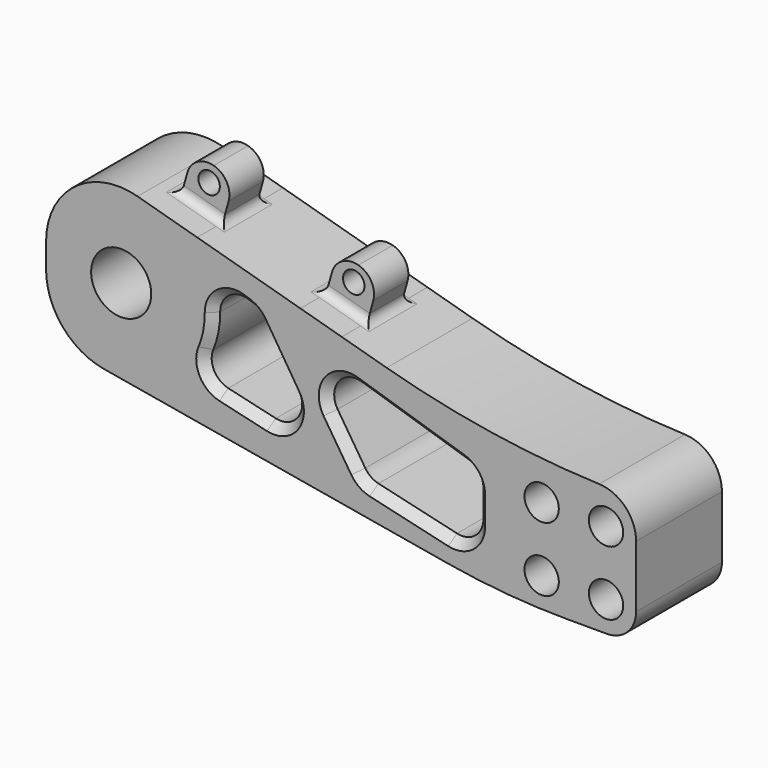
from build123d import *

# Parameters (mm, degrees)
F0_W          = 30
F0_H          = 30
F0_R          = 4
F0_R_2        = 7
F1_DEPTH      = 25
F2_R          = 16.7849194194
F3_R          = 16.2658089237
F4_R          = 212.1999742311
F5_R          = 163.8141108575
F6_R          = 8.9325901808
F7_R          = 6.7597979746
F9_DEPTH      = 25
F10_R         = 5
F11_SIZE      = 2
F13_DEPTH     = 7.5
F15_DEPTH     = 7.5
F16_T1_DEPTH  = 10
F16_T3_DEPTH  = 10
F16_T5_DEPTH  = 10
F16_T7_DEPTH  = 10
F16_T9_DEPTH  = 10
F16_T15_DEPTH = 12
F16_T19_DEPTH = 12
F16_T26_DEPTH = 12
F16_T30_DEPTH = 12
F16_T37_DEPTH = 12
F16_T41_DEPTH = 12
F16_T48_DEPTH = 12
F16_T52_DEPTH = 12
F16_T59_DEPTH = 12
F16_T63_DEPTH = 12
F16_T70_DEPTH = 12
F16_T74_DEPTH = 12
F16_T81_DEPTH = 12
F16_T85_DEPTH = 12
F16_T92_DEPTH = 12
F16_T96_DEPTH = 12
F17_R         = 2.5
F18_DEPTH     = 25
F19_R         = 4.99999


# Not quite as in the source:
# - a fillet or chamfer that OpenCascade refuses, or shapes differently, is made with other operations: its cross-section is extruded or revolved along the edge and cut away or added
# - a fillet or chamfer is up to 0.001 mm smaller than in the source, because OpenCascade refuses the exact size


with BuildPart() as f1:
    # F0 (on Front) → F1 (new body)
    with BuildSketch(Plane.XZ):
        Rectangle(F0_W, F0_H)
        with Locations((-7, -8)):
            Circle(F0_R, mode=Mode.SUBTRACT)
        with Locations((8, -8)):
            Circle(F0_R, mode=Mode.SUBTRACT)
        with Locations((-7, 7)):
            Circle(F0_R, mode=Mode.SUBTRACT)
        with Locations((8, 7)):
            Circle(F0_R, mode=Mode.SUBTRACT)
        Polygon((-15, -15), (-15, 15), (-53.5854479095, 25.8251958423), (-63.2137087554, 28.5264165077), (-87.2843608702, 35.2794681713), (-96.9126217161, 37.9806888367), (-122.4668100476, 45.1499484479), (-122.4668100476, 3.5487897694), align=None)
        with Locations((-104.9668100476, 20.1499484479)):
            Circle(F0_R_2, mode=Mode.SUBTRACT)
        Polygon((-63.2137087554, 28.5264165077), (-53.5854479095, 25.8251958423), (-50.8842272441, 35.4534566882), (-60.51248809, 38.1546773536), align=None)
        Polygon((-96.9126217161, 37.9806888367), (-87.2843608702, 35.2794681713), (-84.5831402048, 44.9077290172), (-94.2114010507, 47.6089496826), align=None)
    extrude(amount=F1_DEPTH)

    # F2
    f2_edges = [f1.edges().sort_by_distance(p)[0] for p in [
        (-122.46681, -12.5, 45.149948),
    ]]
    fillet(f2_edges, radius=F2_R)

    # F3
    f3_edges = [f1.edges().sort_by_distance(p)[0] for p in [
        (-122.46681, -12.5, 3.54879),
    ]]
    fillet(f3_edges, radius=F3_R)

    # F4
    f4_edges = [f1.edges().sort_by_distance(p)[0] for p in [
        (-15, -12.5, 15),
    ]]
    fillet(f4_edges, radius=F4_R)

    # F5
    f5_edges = [f1.edges().sort_by_distance(p)[0] for p in [
        (-15, -12.5, -15),
    ]]
    fillet(f5_edges, radius=F5_R)

    # F6
    f6_edges = [f1.edges().sort_by_distance(p)[0] for p in [
        (15, -12.5, 15),
    ]]
    fillet(f6_edges, radius=F6_R)

    # F7
    f7_edges = [f1.edges().sort_by_distance(p)[0] for p in [
        (15, -12.5, -15),
    ]]
    fillet(f7_edges, radius=F7_R)

    # F8 (on face) → F9 (cut)
    with BuildSketch(Plane.XZ.offset(25)):
        with BuildLine():
            Line((-73.9658618647, 24.2199581794), (-84.8379017791, 27.6423353583))
            ThreePointArc((-84.8379017791, 27.6423353583), (-83.7792374174, 16.8291979096), (-88.2094318459, 6.9086087616))
            Line((-88.2094318459, 6.9086087616), (-58.6424097419, 0))
            Line((-58.6424097419, 0), (-73.9658618647, 24.2199581794))
        make_face()
        Polygon((-22.1739318222, -8.5211978803), (-22.1739318222, 7.9165302277), (-63.6694356799, 20.978776738), (-48.5837496817, -2.3502991535), align=None)
    extrude(amount=-F9_DEPTH, mode=Mode.SUBTRACT)

    # F10
    f10_edges = [f1.edges().sort_by_distance(p)[0] for p in [
        (-88.209432, -12.5, 6.908609),
        (-84.837902, -12.5, 27.642335),
        (-73.965862, -12.5, 24.219958),
        (-58.64241, -12.5, 0),
        (-63.669436, -12.5, 20.978777),
        (-48.58375, -12.5, -2.350299),
        (-22.173932, -12.5, -8.521198),
        (-22.173932, -12.5, 7.91653),
    ]]
    fillet(f10_edges, radius=F10_R)

    # F11
    f11_edges = [f1.edges().sort_by_distance(p)[0] for p in [
        (-81.475167, -25, 24.42871),
        (-38.054326, -25, 12.915472),
        (-38.054326, 0, 12.915472),
        (-69.079861, 0, 16.497238),
        (-52.90778, 0, 4.336545),
        (-55.915109, 0, 15.073198),
        (-48.358225, 0, -2.029785),
        (-37.465092, 0, -4.948277),
        (-23.142397, 0, 7.206075),
        (-24.066543, 0, -6.135382),
        (-22.173932, 0, 1.015182),
        (-76.357367, 0, 24.972773),
        (-74.163675, 0, 23.962872),
        (-81.475167, 0, 24.42871),
        (-83.895301, 0, 16.17939),
        (-65.322794, 0, 4.750228),
        (-84.930719, 0, 7.951227),
        (-76.078695, 0, 4.07415),
        (-52.90778, -25, 4.336545),
        (-55.915109, -25, 15.073198),
        (-48.358225, -25, -2.029785),
        (-37.465092, -25, -4.948277),
        (-23.142397, -25, 7.206075),
        (-24.066543, -25, -6.135382),
        (-22.173932, -25, 1.015182),
        (-76.357367, -25, 24.972773),
        (-74.163675, -25, 23.962872),
        (-69.079861, -25, 16.497238),
        (-83.895301, -25, 16.17939),
        (-65.322794, -25, 4.750228),
        (-84.930719, -25, 7.951227),
        (-76.078695, -25, 4.07415),
    ]]
    chamfer(f11_edges, length=F11_SIZE)

    # F12 (on face) → F13 (cut)
    with BuildSketch(Plane.XZ.offset(25)):
        Polygon((-50.8842272441, 35.4534566882), (-60.51248809, 38.1546773536), (-63.2137087554, 28.5264165077), (-53.5854479095, 25.8251958423), align=None)
        Polygon((-87.2843608702, 35.2794681713), (-84.5831402048, 44.9077290172), (-94.2114010507, 47.6089496826), (-96.9126217161, 37.9806888367), align=None)
    extrude(amount=-F13_DEPTH, mode=Mode.SUBTRACT)

    # F14 (on face) → F15 (cut)
    with BuildSketch(Plane(origin=(0, 0, 0), x_dir=(-1, 0, 0), z_dir=(0, 1, 0))):
        Polygon((53.5854479095, 25.8251958423), (63.2137087554, 28.5264165077), (60.51248809, 38.1546773536), (50.8842272441, 35.4534566882), align=None)
        Polygon((94.2114010507, 47.6089496826), (84.5831402048, 44.9077290172), (87.2843608702, 35.2794681713), (96.9126217161, 37.9806888367), align=None)
    extrude(amount=-F15_DEPTH, mode=Mode.SUBTRACT)

    # F16: fillet of radius 2 on 8 edges, made by hand

    # F16_s2 → F16_t1 (join)
    with BuildSketch(Plane(origin=(-56.3921675224, 0, 15.8208933801), x_dir=(0, 1, 0), z_dir=(-0.9628260846, 0, 0.2701220665))):
        with BuildLine():
            ThreePointArc((-5.5, -10.3905602707), (-6.9142135624, -10.9763467084), (-7.5, -12.3905602707))
            Line((-7.5, -12.3905602707), (-7.54, -12.3905602707))
            Line((-7.54, -12.3905602707), (-7.54, -10.3505602707))
            Line((-7.54, -10.3505602707), (-5.5, -10.3505602707))
            Line((-5.5, -10.3505602707), (-5.5, -10.3905602707))
        make_face()
    extrude(amount=F16_T1_DEPTH)

    # F16_s4 → F16_t3 (join)
    with BuildSketch(Plane.XZ.offset(7.5)):
        with BuildLine():
            ThreePointArc((-51.6597957404, 25.2849517092), (-52.8632036043, 26.2309724614), (-53.0452037765, 27.7508480115))
            Line((-53.0452037765, 27.7508480115), (-53.0837168198, 27.7616528941))
            Line((-53.0837168198, 27.7616528941), (-53.6347658356, 25.7974876816))
            Line((-53.6347658356, 25.7974876816), (-51.670600623, 25.2464386658))
            Line((-51.670600623, 25.2464386658), (-51.6597957404, 25.2849517092))
        make_face()
        with BuildLine():
            ThreePointArc((-65.1393609246, 29.0666606408), (-63.6194853745, 29.248660813), (-62.6734646224, 30.4520686769))
            Line((-62.6734646224, 30.4520686769), (-62.634951579, 30.4412637942))
            Line((-62.634951579, 30.4412637942), (-63.1860005947, 28.4770985817))
            Line((-63.1860005947, 28.4770985817), (-65.1501658073, 29.0281475974))
            Line((-65.1501658073, 29.0281475974), (-65.1393609246, 29.0666606408))
        make_face()
        with BuildLine():
            ThreePointArc((-85.358708701, 34.7392240382), (-86.562116565, 35.6852447903), (-86.7441167371, 37.2051203404))
            Line((-86.7441167371, 37.2051203404), (-86.7826297805, 37.2159252231))
            Line((-86.7826297805, 37.2159252231), (-87.3336787962, 35.2517600105))
            Line((-87.3336787962, 35.2517600105), (-85.3695135837, 34.7007109948))
            Line((-85.3695135837, 34.7007109948), (-85.358708701, 34.7392240382))
        make_face()
        with BuildLine():
            ThreePointArc((-98.8382738853, 38.5209329698), (-97.3183983352, 38.7029331419), (-96.372377583, 39.9063410059))
            Line((-96.372377583, 39.9063410059), (-96.3338645396, 39.8955361232))
            Line((-96.3338645396, 39.8955361232), (-96.8849135554, 37.9313709106))
            Line((-96.8849135554, 37.9313709106), (-98.8490787679, 38.4824199264))
            Line((-98.8490787679, 38.4824199264), (-98.8382738853, 38.5209329698))
        make_face()
    extrude(amount=F16_T3_DEPTH)

    # F16_s6 → F16_t5 (join)
    with BuildSketch(Plane(origin=(-66.0204283683, 0, 18.5221140456), x_dir=(0, 1, 0), z_dir=(0.9628260846, 0, -0.2701220665))):
        with BuildLine():
            ThreePointArc((-19.5, 10.3905602707), (-18.0857864376, 10.9763467084), (-17.5, 12.3905602707))
            Line((-17.5, 12.3905602707), (-17.46, 12.3905602707))
            Line((-17.46, 12.3905602707), (-17.46, 10.3505602707))
            Line((-17.46, 10.3505602707), (-19.5, 10.3505602707))
            Line((-19.5, 10.3505602707), (-19.5, 10.3905602707))
        make_face()
    extrude(amount=F16_T5_DEPTH)

    # F16_s8 → F16_t7 (join)
    with BuildSketch(Plane(origin=(-99.7193413289, 0, 27.9763863745), x_dir=(0, 1, 0), z_dir=(0.9628260846, 0, -0.2701220665))):
        with BuildLine():
            ThreePointArc((-19.5, 10.3905602707), (-18.0857864376, 10.9763467084), (-17.5, 12.3905602707))
            Line((-17.5, 12.3905602707), (-17.46, 12.3905602707))
            Line((-17.46, 12.3905602707), (-17.46, 10.3505602707))
            Line((-17.46, 10.3505602707), (-19.5, 10.3505602707))
            Line((-19.5, 10.3505602707), (-19.5, 10.3905602707))
        make_face()
    extrude(amount=F16_T7_DEPTH)

    # F16_s10 → F16_t9 (join)
    with BuildSketch(Plane(origin=(-90.091080483, 0, 25.2751657091), x_dir=(0, 1, 0), z_dir=(-0.9628260846, 0, 0.2701220665))):
        with BuildLine():
            ThreePointArc((-5.5, -10.3905602707), (-6.9142135624, -10.9763467084), (-7.5, -12.3905602707))
            Line((-7.5, -12.3905602707), (-7.54, -12.3905602707))
            Line((-7.54, -12.3905602707), (-7.54, -10.3505602707))
            Line((-7.54, -10.3505602707), (-5.5, -10.3505602707))
            Line((-5.5, -10.3505602707), (-5.5, -10.3905602707))
        make_face()
    extrude(amount=F16_T9_DEPTH)


with BuildPart() as f16_tool13:
    # F16_s14 → F16_t15 (new body)
    with BuildSketch(Plane.XZ.offset(5.5)):
        with BuildLine():
            ThreePointArc((-51.6597957404, 25.2849517092), (-52.8632036043, 26.2309724614), (-53.0452037765, 27.7508480115))
            Line((-53.0452037765, 27.7508480115), (-53.0837168198, 27.7616528941))
            Line((-53.0837168198, 27.7616528941), (-53.6347658356, 25.7974876816))
            Line((-53.6347658356, 25.7974876816), (-51.670600623, 25.2464386658))
            Line((-51.670600623, 25.2464386658), (-51.6597957404, 25.2849517092))
        make_face()
    extrude(amount=F16_T15_DEPTH)

    split(bisect_by=Plane.XZ.offset(7.5), keep=Keep.BOTTOM)


with BuildPart() as f16_tool17:
    # F16_s18 → F16_t19 (new body)
    with BuildSketch(Plane(origin=(-54.4665153532, 0, 15.2806492471), x_dir=(0, 1, 0), z_dir=(-0.9628260846, 0, 0.2701220665))):
        with BuildLine():
            ThreePointArc((-5.5, -10.3905602707), (-6.9142135624, -10.9763467084), (-7.5, -12.3905602707))
            Line((-7.5, -12.3905602707), (-7.54, -12.3905602707))
            Line((-7.54, -12.3905602707), (-7.54, -10.3505602707))
            Line((-7.54, -10.3505602707), (-5.5, -10.3505602707))
            Line((-5.5, -10.3505602707), (-5.5, -10.3905602707))
        make_face()
    extrude(amount=F16_T19_DEPTH)

    split(bisect_by=Plane(origin=(-56.3921675224, 0, 15.8208933801), x_dir=(0, 1, 0), z_dir=(0.9628260846, 0, -0.2701220665)), keep=Keep.TOP)


with BuildPart() as f16_tool13_1:
    add(f16_tool13.part)

    # F16_t21: intersect F16_tool17
    add(f16_tool17.part, mode=Mode.INTERSECT)


with BuildPart() as f1_1:
    add(f1.part)

    # F16_t11: union F16_tool13
    add(f16_tool13_1.part)


with BuildPart() as f16_tool24:
    # F16_s25 → F16_t26 (new body)
    with BuildSketch(Plane.XZ.offset(5.5)):
        with BuildLine():
            ThreePointArc((-65.1393609246, 29.0666606408), (-63.6194853745, 29.248660813), (-62.6734646224, 30.4520686769))
            Line((-62.6734646224, 30.4520686769), (-62.634951579, 30.4412637942))
            Line((-62.634951579, 30.4412637942), (-63.1860005947, 28.4770985817))
            Line((-63.1860005947, 28.4770985817), (-65.1501658073, 29.0281475974))
            Line((-65.1501658073, 29.0281475974), (-65.1393609246, 29.0666606408))
        make_face()
    extrude(amount=F16_T26_DEPTH)

    split(bisect_by=Plane.XZ.offset(7.5), keep=Keep.BOTTOM)


with BuildPart() as f16_tool28:
    # F16_s29 → F16_t30 (new body)
    with BuildSketch(Plane(origin=(-56.3921675224, 0, 15.8208933801), x_dir=(0, 1, 0), z_dir=(-0.9628260846, 0, 0.2701220665))):
        with BuildLine():
            ThreePointArc((-5.5, -10.3905602707), (-6.9142135624, -10.9763467084), (-7.5, -12.3905602707))
            Line((-7.5, -12.3905602707), (-7.54, -12.3905602707))
            Line((-7.54, -12.3905602707), (-7.54, -10.3505602707))
            Line((-7.54, -10.3505602707), (-5.5, -10.3505602707))
            Line((-5.5, -10.3505602707), (-5.5, -10.3905602707))
        make_face()
    extrude(amount=F16_T30_DEPTH)

    split(bisect_by=Plane(origin=(-66.0204283683, 0, 18.5221140456), x_dir=(0, 1, 0), z_dir=(-0.9628260846, 0, 0.2701220665)), keep=Keep.TOP)


with BuildPart() as f16_tool24_1:
    add(f16_tool24.part)

    # F16_t32: intersect F16_tool28
    add(f16_tool28.part, mode=Mode.INTERSECT)


with BuildPart() as f1_2:
    add(f1_1.part)

    # F16_t22: union F16_tool24
    add(f16_tool24_1.part)


with BuildPart() as f16_tool35:
    # F16_s36 → F16_t37 (new body)
    with BuildSketch(Plane(origin=(-66.0204283683, 0, 18.5221140456), x_dir=(0, 1, 0), z_dir=(0.9628260846, 0, -0.2701220665))):
        with BuildLine():
            ThreePointArc((-19.5, 10.3905602707), (-18.0857864376, 10.9763467084), (-17.5, 12.3905602707))
            Line((-17.5, 12.3905602707), (-17.46, 12.3905602707))
            Line((-17.46, 12.3905602707), (-17.46, 10.3505602707))
            Line((-17.46, 10.3505602707), (-19.5, 10.3505602707))
            Line((-19.5, 10.3505602707), (-19.5, 10.3905602707))
        make_face()
    extrude(amount=F16_T37_DEPTH)

    split(bisect_by=Plane(origin=(-56.3921675224, 0, 15.8208933801), x_dir=(0, 1, 0), z_dir=(0.9628260846, 0, -0.2701220665)), keep=Keep.TOP)


with BuildPart() as f16_tool39:
    # F16_s40 → F16_t41 (new body)
    with BuildSketch(Plane.XZ.offset(7.5)):
        with BuildLine():
            ThreePointArc((-51.6597957404, 25.2849517092), (-52.8632036043, 26.2309724614), (-53.0452037765, 27.7508480115))
            Line((-53.0452037765, 27.7508480115), (-53.0837168198, 27.7616528941))
            Line((-53.0837168198, 27.7616528941), (-53.6347658356, 25.7974876816))
            Line((-53.6347658356, 25.7974876816), (-51.670600623, 25.2464386658))
            Line((-51.670600623, 25.2464386658), (-51.6597957404, 25.2849517092))
        make_face()
    extrude(amount=F16_T41_DEPTH)

    split(bisect_by=Plane.XZ.offset(17.5), keep=Keep.TOP)


with BuildPart() as f16_tool35_1:
    add(f16_tool35.part)

    # F16_t43: intersect F16_tool39
    add(f16_tool39.part, mode=Mode.INTERSECT)


with BuildPart() as f1_3:
    add(f1_2.part)

    # F16_t33: union F16_tool35
    add(f16_tool35_1.part)


with BuildPart() as f16_tool46:
    # F16_s47 → F16_t48 (new body)
    with BuildSketch(Plane.XZ.offset(7.5)):
        with BuildLine():
            ThreePointArc((-65.1393609246, 29.0666606408), (-63.6194853745, 29.248660813), (-62.6734646224, 30.4520686769))
            Line((-62.6734646224, 30.4520686769), (-62.634951579, 30.4412637942))
            Line((-62.634951579, 30.4412637942), (-63.1860005947, 28.4770985817))
            Line((-63.1860005947, 28.4770985817), (-65.1501658073, 29.0281475974))
            Line((-65.1501658073, 29.0281475974), (-65.1393609246, 29.0666606408))
        make_face()
    extrude(amount=F16_T48_DEPTH)

    split(bisect_by=Plane.XZ.offset(17.5), keep=Keep.TOP)


with BuildPart() as f16_tool50:
    # F16_s51 → F16_t52 (new body)
    with BuildSketch(Plane(origin=(-67.9460805375, 0, 19.0623581786), x_dir=(0, 1, 0), z_dir=(0.9628260846, 0, -0.2701220665))):
        with BuildLine():
            ThreePointArc((-19.5, 10.3905602707), (-18.0857864376, 10.9763467084), (-17.5, 12.3905602707))
            Line((-17.5, 12.3905602707), (-17.46, 12.3905602707))
            Line((-17.46, 12.3905602707), (-17.46, 10.3505602707))
            Line((-17.46, 10.3505602707), (-19.5, 10.3505602707))
            Line((-19.5, 10.3505602707), (-19.5, 10.3905602707))
        make_face()
    extrude(amount=F16_T52_DEPTH)

    split(bisect_by=Plane(origin=(-66.0204283683, 0, 18.5221140456), x_dir=(0, 1, 0), z_dir=(-0.9628260846, 0, 0.2701220665)), keep=Keep.TOP)


with BuildPart() as f16_tool46_1:
    add(f16_tool46.part)

    # F16_t54: intersect F16_tool50
    add(f16_tool50.part, mode=Mode.INTERSECT)


with BuildPart() as f1_4:
    add(f1_3.part)

    # F16_t44: union F16_tool46
    add(f16_tool46_1.part)


with BuildPart() as f16_tool57:
    # F16_s58 → F16_t59 (new body)
    with BuildSketch(Plane.XZ.offset(5.5)):
        with BuildLine():
            ThreePointArc((-85.358708701, 34.7392240382), (-86.562116565, 35.6852447903), (-86.7441167371, 37.2051203404))
            Line((-86.7441167371, 37.2051203404), (-86.7826297805, 37.2159252231))
            Line((-86.7826297805, 37.2159252231), (-87.3336787962, 35.2517600105))
            Line((-87.3336787962, 35.2517600105), (-85.3695135837, 34.7007109948))
            Line((-85.3695135837, 34.7007109948), (-85.358708701, 34.7392240382))
        make_face()
    extrude(amount=F16_T59_DEPTH)

    split(bisect_by=Plane.XZ.offset(7.5), keep=Keep.BOTTOM)


with BuildPart() as f16_tool61:
    # F16_s62 → F16_t63 (new body)
    with BuildSketch(Plane(origin=(-88.1654283139, 0, 24.734921576), x_dir=(0, 1, 0), z_dir=(-0.9628260846, 0, 0.2701220665))):
        with BuildLine():
            ThreePointArc((-5.5, -10.3905602707), (-6.9142135624, -10.9763467084), (-7.5, -12.3905602707))
            Line((-7.5, -12.3905602707), (-7.54, -12.3905602707))
            Line((-7.54, -12.3905602707), (-7.54, -10.3505602707))
            Line((-7.54, -10.3505602707), (-5.5, -10.3505602707))
            Line((-5.5, -10.3505602707), (-5.5, -10.3905602707))
        make_face()
    extrude(amount=F16_T63_DEPTH)

    split(bisect_by=Plane(origin=(-90.091080483, 0, 25.2751657091), x_dir=(0, 1, 0), z_dir=(0.9628260846, 0, -0.2701220665)), keep=Keep.TOP)


with BuildPart() as f16_tool57_1:
    add(f16_tool57.part)

    # F16_t65: intersect F16_tool61
    add(f16_tool61.part, mode=Mode.INTERSECT)


with BuildPart() as f1_5:
    add(f1_4.part)

    # F16_t55: union F16_tool57
    add(f16_tool57_1.part)


with BuildPart() as f16_tool68:
    # F16_s69 → F16_t70 (new body)
    with BuildSketch(Plane(origin=(-99.7193413289, 0, 27.9763863745), x_dir=(0, 1, 0), z_dir=(0.9628260846, 0, -0.2701220665))):
        with BuildLine():
            ThreePointArc((-19.5, 10.3905602707), (-18.0857864376, 10.9763467084), (-17.5, 12.3905602707))
            Line((-17.5, 12.3905602707), (-17.46, 12.3905602707))
            Line((-17.46, 12.3905602707), (-17.46, 10.3505602707))
            Line((-17.46, 10.3505602707), (-19.5, 10.3505602707))
            Line((-19.5, 10.3505602707), (-19.5, 10.3905602707))
        make_face()
    extrude(amount=F16_T70_DEPTH)

    split(bisect_by=Plane(origin=(-90.091080483, 0, 25.2751657091), x_dir=(0, 1, 0), z_dir=(0.9628260846, 0, -0.2701220665)), keep=Keep.TOP)


with BuildPart() as f16_tool72:
    # F16_s73 → F16_t74 (new body)
    with BuildSketch(Plane.XZ.offset(7.5)):
        with BuildLine():
            ThreePointArc((-85.358708701, 34.7392240382), (-86.562116565, 35.6852447903), (-86.7441167371, 37.2051203404))
            Line((-86.7441167371, 37.2051203404), (-86.7826297805, 37.2159252231))
            Line((-86.7826297805, 37.2159252231), (-87.3336787962, 35.2517600105))
            Line((-87.3336787962, 35.2517600105), (-85.3695135837, 34.7007109948))
            Line((-85.3695135837, 34.7007109948), (-85.358708701, 34.7392240382))
        make_face()
    extrude(amount=F16_T74_DEPTH)

    split(bisect_by=Plane.XZ.offset(17.5), keep=Keep.TOP)


with BuildPart() as f16_tool68_1:
    add(f16_tool68.part)

    # F16_t76: intersect F16_tool72
    add(f16_tool72.part, mode=Mode.INTERSECT)


with BuildPart() as f1_6:
    add(f1_5.part)

    # F16_t66: union F16_tool68
    add(f16_tool68_1.part)


with BuildPart() as f16_tool79:
    # F16_s80 → F16_t81 (new body)
    with BuildSketch(Plane.XZ.offset(7.5)):
        with BuildLine():
            ThreePointArc((-98.8382738853, 38.5209329698), (-97.3183983352, 38.7029331419), (-96.372377583, 39.9063410059))
            Line((-96.372377583, 39.9063410059), (-96.3338645396, 39.8955361232))
            Line((-96.3338645396, 39.8955361232), (-96.8849135554, 37.9313709106))
            Line((-96.8849135554, 37.9313709106), (-98.8490787679, 38.4824199264))
            Line((-98.8490787679, 38.4824199264), (-98.8382738853, 38.5209329698))
        make_face()
    extrude(amount=F16_T81_DEPTH)

    split(bisect_by=Plane.XZ.offset(17.5), keep=Keep.TOP)


with BuildPart() as f16_tool83:
    # F16_s84 → F16_t85 (new body)
    with BuildSketch(Plane(origin=(-101.6449934981, 0, 28.5166305076), x_dir=(0, 1, 0), z_dir=(0.9628260846, 0, -0.2701220665))):
        with BuildLine():
            ThreePointArc((-19.5, 10.3905602707), (-18.0857864376, 10.9763467084), (-17.5, 12.3905602707))
            Line((-17.5, 12.3905602707), (-17.46, 12.3905602707))
            Line((-17.46, 12.3905602707), (-17.46, 10.3505602707))
            Line((-17.46, 10.3505602707), (-19.5, 10.3505602707))
            Line((-19.5, 10.3505602707), (-19.5, 10.3905602707))
        make_face()
    extrude(amount=F16_T85_DEPTH)

    split(bisect_by=Plane(origin=(-99.7193413289, 0, 27.9763863745), x_dir=(0, 1, 0), z_dir=(-0.9628260846, 0, 0.2701220665)), keep=Keep.TOP)


with BuildPart() as f16_tool79_1:
    add(f16_tool79.part)

    # F16_t87: intersect F16_tool83
    add(f16_tool83.part, mode=Mode.INTERSECT)


with BuildPart() as f1_7:
    add(f1_6.part)

    # F16_t77: union F16_tool79
    add(f16_tool79_1.part)


with BuildPart() as f16_tool90:
    # F16_s91 → F16_t92 (new body)
    with BuildSketch(Plane.XZ.offset(5.5)):
        with BuildLine():
            ThreePointArc((-98.8382738853, 38.5209329698), (-97.3183983352, 38.7029331419), (-96.372377583, 39.9063410059))
            Line((-96.372377583, 39.9063410059), (-96.3338645396, 39.8955361232))
            Line((-96.3338645396, 39.8955361232), (-96.8849135554, 37.9313709106))
            Line((-96.8849135554, 37.9313709106), (-98.8490787679, 38.4824199264))
            Line((-98.8490787679, 38.4824199264), (-98.8382738853, 38.5209329698))
        make_face()
    extrude(amount=F16_T92_DEPTH)

    split(bisect_by=Plane.XZ.offset(7.5), keep=Keep.BOTTOM)


with BuildPart() as f16_tool94:
    # F16_s95 → F16_t96 (new body)
    with BuildSketch(Plane(origin=(-90.091080483, 0, 25.2751657091), x_dir=(0, 1, 0), z_dir=(-0.9628260846, 0, 0.2701220665))):
        with BuildLine():
            ThreePointArc((-5.5, -10.3905602707), (-6.9142135624, -10.9763467084), (-7.5, -12.3905602707))
            Line((-7.5, -12.3905602707), (-7.54, -12.3905602707))
            Line((-7.54, -12.3905602707), (-7.54, -10.3505602707))
            Line((-7.54, -10.3505602707), (-5.5, -10.3505602707))
            Line((-5.5, -10.3505602707), (-5.5, -10.3905602707))
        make_face()
    extrude(amount=F16_T96_DEPTH)

    split(bisect_by=Plane(origin=(-99.7193413289, 0, 27.9763863745), x_dir=(0, 1, 0), z_dir=(-0.9628260846, 0, 0.2701220665)), keep=Keep.TOP)


with BuildPart() as f16_tool90_1:
    add(f16_tool90.part)

    # F16_t98: intersect F16_tool94
    add(f16_tool94.part, mode=Mode.INTERSECT)


with BuildPart() as f1_8:
    add(f1_7.part)

    # F16_t88: union F16_tool90
    add(f16_tool90_1.part)

    # F17 (on face) → F18 (cut)
    with BuildSketch(Plane(origin=(0, -7.5, 0), x_dir=(-1, 0, 0), z_dir=(0, 1, 0))):
        with Locations((56.7788459332, 32.9527626826)):
            Circle(F17_R)
        with Locations((90.4777588939, 42.4070350115)):
            Circle(F17_R)
    extrude(amount=-F18_DEPTH, mode=Mode.SUBTRACT)

    # F19 (radius 5 in the source; OpenCascade refuses exactly that, so slightly less here)
    f19_edges = [f1_8.edges().sort_by_distance(p)[0] for p in [
        (-84.58314, -12.5, 44.907729),
        (-94.211401, -12.5, 47.60895),
        (-50.884227, -12.5, 35.453457),
        (-60.512488, -12.5, 38.154677),
    ]]
    fillet(f19_edges, radius=F19_R)


solid = f1_8.part
